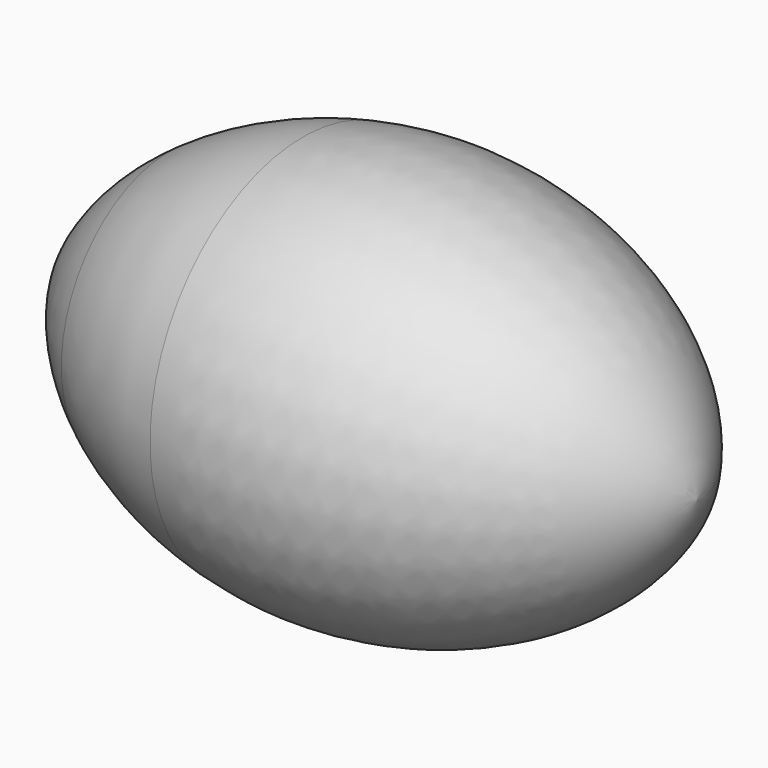
from build123d import *


with BuildPart() as f1:
    # F0 (on Top) → F1 (revolve)
    with BuildSketch(Plane.XY):
        with BuildLine():
            add(Edge.make_bspline(
                [(-81.9881628618, 51.4834874052), (-87.8374344249, 47.4250360241), (-103.2349607209, 34.5172153184), (-117.5591673418, 12.4343589375), (-119.0711009096, 3.3734235422), (-119.634, 0)],
                knots=[0.7436766169, 0.7436766169, 0.7436766169, 0.7436766169, 0.8078231103, 0.928451753, 1, 1, 1, 1], degree=3))
            Line((-119.634, 0), (-46.3161534692, 0))
            ThreePointArc((-46.3161534692, 0), (-77.6332482946, 16.4009317657), (-81.9881628618, 51.4834874052))
        make_face()
        with BuildLine():
            ThreePointArc((-8.2161533182, 38.1), (-19.3753850084, 11.1592315834), (-46.3161534692, 0))
            Line((-46.3161534692, 0), (119.634, 0))
            add(Edge.make_bspline(
                [(119.634, 0), (119.0711009096, 3.3734235422), (117.5591673418, 12.4343589375), (98.573454101, 41.7036085289), (57.5611036651, 68.4820593391), (9.2823174411, 78.3256138413), (-20.8506096484, 75.0755532283), (-30.9393429568, 72.9591982568)],
                knots=[0, 0, 0, 0, 0.071548247, 0.1921768897, 0.3397383448, 0.5, 0.5847781931, 0.5847781931, 0.5847781931, 0.5847781931], degree=3))
            ThreePointArc((-30.9393429568, 72.9591982568), (-14.3985525722, 58.9056906305), (-8.2161533182, 38.1))
        make_face()
        with BuildLine():
            ThreePointArc((-81.9881628618, 51.4834874052), (-77.6332482946, 16.4009317657), (-46.3161534692, 0))
            ThreePointArc((-46.3161534692, 0), (-19.3753850084, 11.1592315834), (-8.2161533182, 38.1))
            ThreePointArc((-8.2161533182, 38.1), (-14.3985525722, 58.9056906305), (-30.9393429568, 72.9591982568))
            add(Edge.make_bspline(
                [(-30.9393429568, 72.9591982568), (-39.9219891935, 71.0748717077), (-58.2694731501, 65.4529293108), (-74.3818739183, 56.7610255626), (-81.9881628618, 51.4834874052)],
                knots=[0.5847781931, 0.5847781931, 0.5847781931, 0.5847781931, 0.6602616552, 0.7436766169, 0.7436766169, 0.7436766169, 0.7436766169], degree=3))
        make_face()
    revolve(axis=Axis((-33.5799832898, 0, 0), (1, 0, 0)))


solid = f1.part
